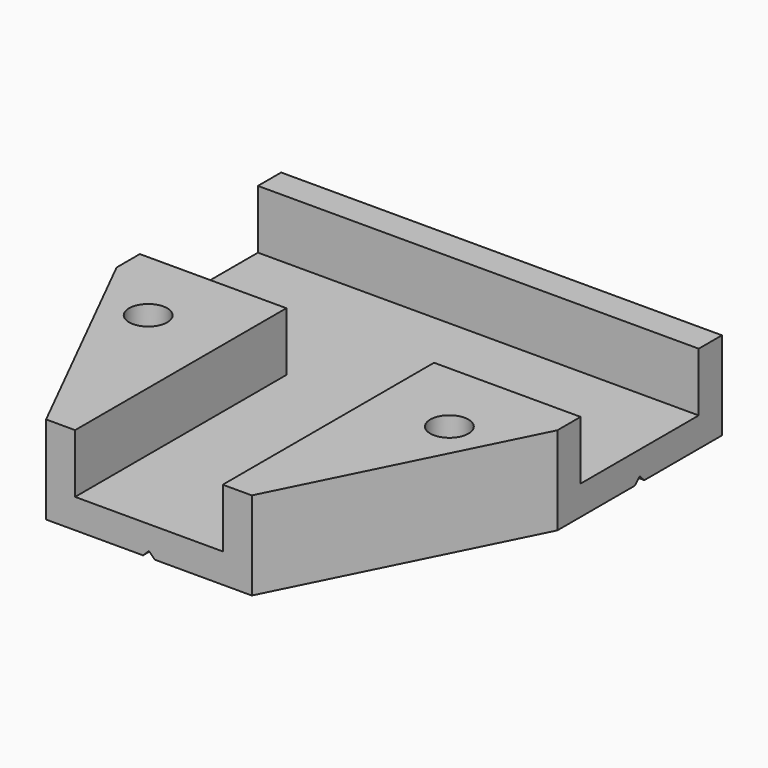
from build123d import *

# Parameters (mm, degrees)
F0_R     = 2.6
F1_DEPTH = 12
F3_W     = 20.1
F3_H     = 8
F4_DEPTH = 30.001
F2_W     = 10.05
F2_H     = 8
F5_DEPTH = 46.001
F7_DEPTH = 5


# Not quite as in the source:
# - a fillet or chamfer that OpenCascade refuses, or shapes differently, is made with other operations: its cross-section is extruded or revolved along the edge and cut away or added


with BuildPart() as f1:
    # F0 (on Top) → F1 (new body)
    with BuildSketch(Plane.XY):
        Polygon((0, -46), (0, 14), (-30, 14), (-30, -14), (-14, -46), align=None)
        with Locations((-20.5, -20.5)):
            Circle(F0_R, mode=Mode.SUBTRACT)
    extrude(amount=F1_DEPTH)

    # F3 (on face) → F4 (cut, through all)
    with BuildSketch(Plane(origin=(-30, 0, 0), x_dir=(0, -1, 0), z_dir=(-1, 0, 0))):
        with Locations((0, 8)):
            Rectangle(F3_W, F3_H)
        Polygon((0, 0.8), (-0.8, 0), (0.8, 0), align=None)
    extrude(amount=-F4_DEPTH, mode=Mode.SUBTRACT)

    # F2 (on face) → F5 (cut, through all)
    with BuildSketch(Plane.XZ.offset(46)):
        with Locations((-5.025, 8)):
            Rectangle(F2_W, F2_H)
        Polygon((-0.8, 0), (0, 0), (0, 0.8), align=None)
    extrude(amount=-F5_DEPTH, mode=Mode.SUBTRACT)

    # F6 (on face) → F7 (cut)
    with BuildSketch(Plane.XY):
        Polygon((-15.9270442062, -21.725319812), (-17.1523640182, -17.1523640182), (-21.725319812, -15.9270442062), (-25.0729557938, -19.274680188), (-23.8476359818, -23.8476359818), (-19.274680188, -25.0729557938), align=None)
    extrude(amount=F7_DEPTH, mode=Mode.SUBTRACT)

    # F8: F1 across plane


with BuildPart() as f1_1:
    add(f1.part)
    add(f1.part.mirror(Plane.YZ))

    # F9: chamfer of 2 on 2 edges, made by hand


with BuildPart() as f9_tool2:
    # F9_s3 → F9_t4 (revolve)
    with BuildSketch(Plane.XZ.offset(20.5)):
        Polygon((17.9, 7), (15.9, 5), (17.9, 5), align=None)
    revolve(axis=Axis((20.5, -20.5, 5), (0, 0, 1)))

    split(bisect_by=Plane(origin=(20.291464501, -5.4370815263, 0), x_dir=(0, 0, 1), z_dir=(0.9659258263, -0.2588190451, 0)), keep=Keep.TOP)

    split(bisect_by=Plane(origin=(-2.8991378029, -2.8991378029, 0), x_dir=(0, 0, 1), z_dir=(0.7071067812, 0.7071067812, 0)), keep=Keep.TOP)

    split(bisect_by=Plane(origin=(5.4370815263, -20.291464501, 0), x_dir=(0, 0, 1), z_dir=(0.2588190451, -0.9659258263, 0)), keep=Keep.TOP)

    split(bisect_by=Plane(origin=(7.5593976961, -28.2120562766, 0), x_dir=(0, 0, 1), z_dir=(-0.2588190451, 0.9659258263, 0)), keep=Keep.TOP)

    split(bisect_by=Plane(origin=(2.8991378029, 2.8991378029, 0), x_dir=(0, 0, 1), z_dir=(-0.7071067812, -0.7071067812, 0)), keep=Keep.TOP)

    split(bisect_by=Plane(origin=(28.2120562766, -7.5593976961, 0), x_dir=(0, 0, 1), z_dir=(-0.9659258263, 0.2588190451, 0)), keep=Keep.TOP)


with BuildPart() as f1_2:
    add(f1_1.part)

    # F9_t1: cut F9_tool2
    add(f9_tool2.part, mode=Mode.SUBTRACT)


with BuildPart() as f9_tool12:
    # F9_s13 → F9_t14 (revolve)
    with BuildSketch(Plane.XZ.offset(20.5)):
        Polygon((-17.9, 7), (-15.9, 5), (-17.9, 5), align=None)
    revolve(axis=Axis((-20.5, -20.5, 5), (0, 0, -1)))

    split(bisect_by=Plane(origin=(-20.291464501, -5.4370815263, 0), x_dir=(0, 0, 1), z_dir=(-0.9659258263, -0.2588190451, 0)), keep=Keep.TOP)

    split(bisect_by=Plane(origin=(2.8991378029, -2.8991378029, 0), x_dir=(0, 0, 1), z_dir=(-0.7071067812, 0.7071067812, 0)), keep=Keep.TOP)

    split(bisect_by=Plane(origin=(-5.4370815263, -20.291464501, 0), x_dir=(0, 0, 1), z_dir=(-0.2588190451, -0.9659258263, 0)), keep=Keep.TOP)

    split(bisect_by=Plane(origin=(-7.5593976961, -28.2120562766, 0), x_dir=(0, 0, 1), z_dir=(0.2588190451, 0.9659258263, 0)), keep=Keep.TOP)

    split(bisect_by=Plane(origin=(-2.8991378029, 2.8991378029, 0), x_dir=(0, 0, 1), z_dir=(0.7071067812, -0.7071067812, 0)), keep=Keep.TOP)

    split(bisect_by=Plane(origin=(-28.2120562766, -7.5593976961, 0), x_dir=(0, 0, 1), z_dir=(0.9659258263, 0.2588190451, 0)), keep=Keep.TOP)


with BuildPart() as f1_3:
    add(f1_2.part)

    # F9_t11: cut F9_tool12
    add(f9_tool12.part, mode=Mode.SUBTRACT)


solid = f1_3.part
